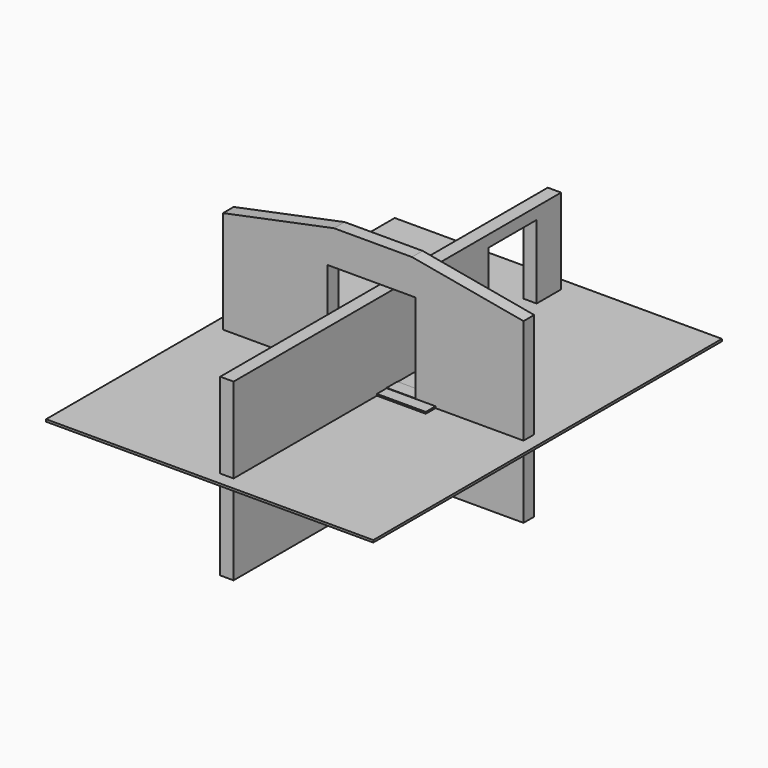
from build123d import *

# Parameters (mm, degrees)
F0_W     = 3740.15
F0_H     = 4981.575
F1_DEPTH = 25.4
F2_W     = 4679.95
F2_H     = 2000.25
F2_W_2   = 688.975
F2_H_2   = 1016
F3_DEPTH = 152.4
F5_DEPTH = 152.4
F6_W     = 1006.475
F6_H     = 1016
F7_DEPTH = 152.4
F8_W     = 1422.4
F8_H     = 584.2
F9_DEPTH = 44.45


# Not quite as in the source:
# - a feature names something its author has since deleted; it is built from what else it names


with BuildPart() as f1:
    # F0 (on Top) → F1 (new body)
    with BuildSketch(Plane.XY):
        Rectangle(F0_W, F0_H)
    extrude(amount=F1_DEPTH)


with BuildPart() as f3:
    # F2 (on Right) → F3 (new body)
    with BuildSketch(Plane.YZ):
        Rectangle(F2_W, F2_H)
        with Locations((1646.0432527542, 358.775)):
            Rectangle(F2_W_2, F2_H_2, mode=Mode.SUBTRACT)
    extrude(amount=F3_DEPTH)


with BuildPart() as f5:
    # F4 (on Front) → F5 (new body)
    with BuildSketch(Plane.XZ):
        Polygon((-1718.6389747441, -802.0838088955), (1716.7110252559, -802.0838088955), (1716.7110252559, 1228.1581670422), (441.9575821344, 1458.5161911045), (-449.6712692842, 1458.5161911045), (-1718.6389747441, 1198.1661911045), align=None)
    extrude(amount=F5_DEPTH)

    # F6 (on face) → F7 (cut)
    with BuildSketch(Plane(origin=(0, 0, 0), x_dir=(-1, 0, 0), z_dir=(0, 1, 0))):
        with Locations((18.4264747441, 556.8161911045)):
            Rectangle(F6_W, F6_H)
    extrude(amount=-F7_DEPTH, mode=Mode.SUBTRACT)


with BuildPart() as f9:
    # F8 (on Top) → F9 (new body)
    with BuildSketch(Plane.XY):
        Rectangle(F8_W, F8_H)
    extrude(amount=F9_DEPTH)


solid = Compound([f1.part, f3.part, f5.part, f9.part])
